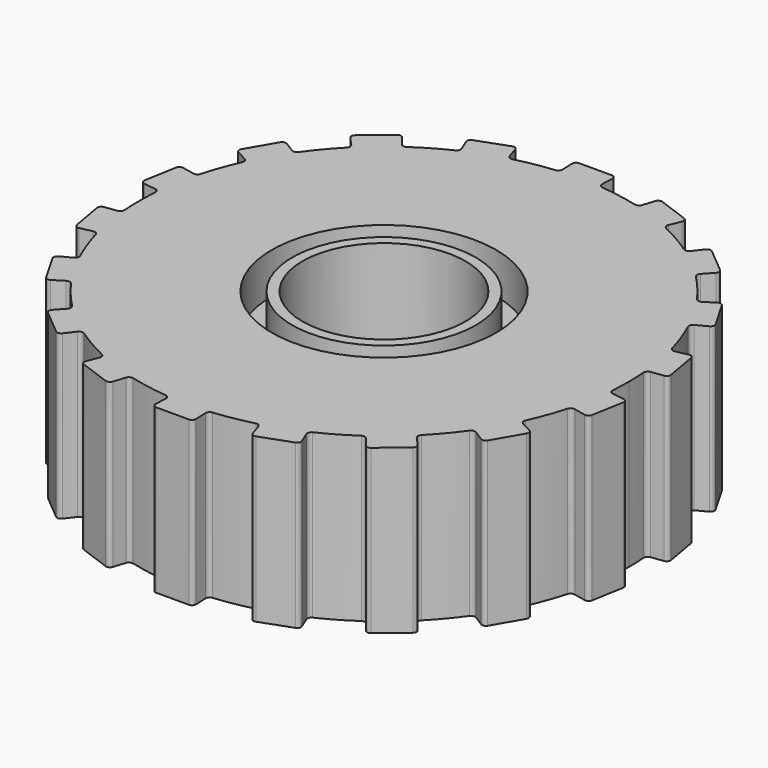
from build123d import *

# Parameters (mm, degrees)
F0_W     = 2.25
F0_H     = 2
F3_DEPTH = 25
F5_R     = 1.375
F5_R_2   = 1.125
F6_DEPTH = 0.5
F4_R     = 1.375
F4_R_2   = 1.125
F7_DEPTH = 0.5


with BuildPart() as f1:
    # F0 (on Front) → F1 (revolve)
    with BuildSketch(Plane.XZ):
        with Locations((-2.125, 1)):
            Rectangle(F0_W, F0_H)
    revolve(axis=Axis((0, 0, 1), (0, 0, 1)))

    # F2 (on face) → F3 (cut)
    with BuildSketch(Plane.XY.offset(2)):
        with BuildLine():
            Line((-0.2480712081, 3.1903703492), (-0.25, 3.2403703492))
            ThreePointArc((-0.25, 3.2403703492), (-0.5643565774, 3.2006251973), (-0.8733487761, 3.1304571416))
            Line((-0.8733487761, 3.1304571416), (-0.8580602404, 3.0828128249))
            Line((-0.8580602404, 3.0828128249), (-0.8121919363, 2.9398714697))
            ThreePointArc((-0.8121919363, 2.9398714697), (-0.7887137207, 2.9105413826), (-0.7516649064, 2.9043071237))
            ThreePointArc((-0.7516649064, 2.9043071237), (-0.520944533, 2.954423259), (-0.2869975729, 2.9862405116))
            Line((-0.2869975729, 2.9862405116), (-0.2980712081, 3.1903703492))
            Line((-0.2980712081, 3.1903703492), (-0.2480712081, 3.1903703492))
        make_face()
        with BuildLine():
            Line((-0.2422844922, 3.0403615286), (-0.2480712081, 3.1903703492))
            Line((-0.2480712081, 3.1903703492), (-0.2980712081, 3.1903703492))
            Line((-0.2980712081, 3.1903703492), (-0.2869975729, 2.9862405116))
            ThreePointArc((-0.2869975729, 2.9862405116), (-0.2543153176, 3.0047702395), (-0.2422844922, 3.0403615286))
        make_face()
        with BuildLine():
            ThreePointArc((-0.2480712081, 3.1903703492), (-0.2346801134, 3.2256042376), (-0.2, 3.2403703492))
            Line((-0.2, 3.2403703492), (-0.25, 3.2403703492))
            Line((-0.25, 3.2403703492), (-0.2480712081, 3.1903703492))
        make_face()
        with BuildLine():
            Line((-0.2, 3.2403703492), (0, 3.2403703492))
            Line((0, 3.2403703492), (0, 3.25))
            ThreePointArc((0, 3.25), (-0.1250926958, 3.247591695), (-0.25, 3.2403703492))
            Line((-0.25, 3.2403703492), (-0.2, 3.2403703492))
        make_face()
        with BuildLine():
            Line((0, 3.25), (0, 3.2403703492))
            Line((0, 3.2403703492), (0.2, 3.2403703492))
            Line((0.2, 3.2403703492), (0.25, 3.2403703492))
            ThreePointArc((0.25, 3.2403703492), (0.1250926958, 3.247591695), (0, 3.25))
        make_face()
        with BuildLine():
            Line((0.25, 3.2403703492), (0.2, 3.2403703492))
            ThreePointArc((0.2, 3.2403703492), (0.2346801134, 3.2256042376), (0.2480712081, 3.1903703492))
            Line((0.2480712081, 3.1903703492), (0.25, 3.2403703492))
        make_face()
        with BuildLine():
            ThreePointArc((0.8733487761, 3.1304571416), (0.5643565774, 3.2006251973), (0.25, 3.2403703492))
            Line((0.25, 3.2403703492), (0.2480712081, 3.1903703492))
            Line((0.2480712081, 3.1903703492), (0.2980712081, 3.1903703492))
            Line((0.2980712081, 3.1903703492), (0.2869975729, 2.9862405116))
            ThreePointArc((0.2869975729, 2.9862405116), (0.520944533, 2.954423259), (0.7516649064, 2.9043071237))
            ThreePointArc((0.7516649064, 2.9043071237), (0.7887137207, 2.9105413826), (0.8121919363, 2.9398714697))
            Line((0.8121919363, 2.9398714697), (0.8580602404, 3.0828128249))
            Line((0.8580602404, 3.0828128249), (0.8733487761, 3.1304571416))
        make_face()
        with BuildLine():
            Line((0.2980712081, 3.1903703492), (0.2480712081, 3.1903703492))
            Line((0.2480712081, 3.1903703492), (0.2422844922, 3.0403615286))
            ThreePointArc((0.2422844922, 3.0403615286), (0.2543153176, 3.0047702395), (0.2869975729, 2.9862405116))
            Line((0.2869975729, 2.9862405116), (0.2980712081, 3.1903703492))
        make_face()
        with BuildLine():
            Line((-1.9296610226, -2.6108252216), (-1.8913588005, -2.6429646021))
            Line((-1.8913588005, -2.6429646021), (-1.8606969603, -2.6034225764))
            ThreePointArc((-1.8606969603, -2.6034225764), (-1.893603041, -2.6218056711), (-1.9296610226, -2.6108252216))
        make_face()
        with BuildLine():
            Line((-2.2360787999, -2.3537101777), (-2.274381022, -2.3215707972))
            ThreePointArc((-2.274381022, -2.3215707972), (-2.0890597315, -2.4896444401), (-1.8913588005, -2.6429646021))
            Line((-1.8913588005, -2.6429646021), (-1.9296610226, -2.6108252216))
            Line((-1.9296610226, -2.6108252216), (-2.2360787999, -2.3537101777))
        make_face()
        with BuildLine():
            Line((-2.2407641013, -2.2845083786), (-2.274381022, -2.3215707972))
            Line((-2.274381022, -2.3215707972), (-2.2360787999, -2.3537101777))
            ThreePointArc((-2.2360787999, -2.3537101777), (-2.2531538345, -2.3201067328), (-2.2407641013, -2.2845083786))
        make_face()
        with BuildLine():
            Line((-2.6389061658, -1.8100211428), (-2.6812430401, -1.8366915255))
            ThreePointArc((-2.6812430401, -1.8366915255), (-2.4896444401, -2.0890597315), (-2.274381022, -2.3215707972))
            Line((-2.274381022, -2.3215707972), (-2.2407641013, -2.2845083786))
            Line((-2.2407641013, -2.2845083786), (-2.1399074085, -2.1733145845))
            ThreePointArc((-2.1399074085, -2.1733145845), (-2.1262459157, -2.1383168097), (-2.1393712963, -2.1031144659))
            ThreePointArc((-2.1393712963, -2.1031144659), (-2.2981333294, -1.9283628291), (-2.4426613584, -1.7416674447))
            ThreePointArc((-2.4426613584, -1.7416674447), (-2.4750497011, -1.7226286454), (-2.5118880744, -1.7300052895))
            Line((-2.5118880744, -1.7300052895), (-2.6389061658, -1.8100211428))
        make_face()
        with BuildLine():
            Line((-2.7062430401, -1.7933902554), (-2.6812430401, -1.8366915255))
            Line((-2.6812430401, -1.8366915255), (-2.6389061658, -1.8100211428))
            ThreePointArc((-2.6389061658, -1.8100211428), (-2.6761151557, -1.8160410588), (-2.7062430401, -1.7933902554))
        make_face()
        with BuildLine():
            Line((-2.9062430401, -1.4469800938), (-2.9312430401, -1.4036788237))
            ThreePointArc((-2.9312430401, -1.4036788237), (-2.8145825623, -1.625), (-2.6812430401, -1.8366915255))
            Line((-2.6812430401, -1.8366915255), (-2.7062430401, -1.7933902554))
            Line((-2.7062430401, -1.7933902554), (-2.9062430401, -1.4469800938))
        make_face()
        with BuildLine():
            Line((-3.0988243417, -0.7983044463), (-3.1477297981, -0.8088863444))
            ThreePointArc((-3.1477297981, -0.8088863444), (-3.0540010176, -1.1115654658), (-2.9312430401, -1.4036788237))
            Line((-2.9312430401, -1.4036788237), (-2.886977374, -1.3803492064))
            Line((-2.886977374, -1.3803492064), (-2.7541725666, -1.3103562391))
            ThreePointArc((-2.7541725666, -1.3103562391), (-2.7293650187, -1.2821415941), (-2.7296589313, -1.2445730669))
            ThreePointArc((-2.7296589313, -1.2445730669), (-2.8190778624, -1.02606043), (-2.8910362027, -0.8011926578))
            ThreePointArc((-2.8910362027, -0.8011926578), (-2.9149596364, -0.7722245729), (-2.9520993448, -0.7665568853))
            Line((-2.9520993448, -0.7665568853), (-3.0988243417, -0.7983044463))
        make_face()
        with BuildLine():
            Line((-2.886977374, -1.3803492064), (-2.9312430401, -1.4036788237))
            Line((-2.9312430401, -1.4036788237), (-2.9062430401, -1.4469800938))
            ThreePointArc((-2.9062430401, -1.4469800938), (-2.910795269, -1.4095631789), (-2.886977374, -1.3803492064))
        make_face()
        with BuildLine():
            Line((-3.2258714781, -0.3657228555), (-3.2345538869, -0.3164824679))
            ThreePointArc((-3.2345538869, -0.3164824679), (-3.2006251973, -0.5643565774), (-3.1477297981, -0.8088863444))
            Line((-3.1477297981, -0.8088863444), (-3.156412207, -0.7596459567))
            Line((-3.156412207, -0.7596459567), (-3.2258714781, -0.3657228555))
        make_face()
        with BuildLine():
            Line((-3.156412207, -0.7596459567), (-3.1477297981, -0.8088863444))
            Line((-3.1477297981, -0.8088863444), (-3.0988243417, -0.7983044463))
            ThreePointArc((-3.0988243417, -0.7983044463), (-3.1358482874, -0.7912350929), (-3.156412207, -0.7596459567))
        make_face()
        with BuildLine():
            Line((-3.1849785681, -0.3096995482), (-3.2345538869, -0.3164824679))
            Line((-3.2345538869, -0.3164824679), (-3.2258714781, -0.3657228555))
            ThreePointArc((-3.2258714781, -0.3657228555), (-3.2173518354, -0.3290055026), (-3.1849785681, -0.3096995482))
        make_face()
        with BuildLine():
            Line((-3.1849785681, 0.3096995482), (-3.2345538869, 0.3164824679))
            ThreePointArc((-3.2345538869, 0.3164824679), (-3.25, 0), (-3.2345538869, -0.3164824679))
            Line((-3.2345538869, -0.3164824679), (-3.1849785681, -0.3096995482))
            Line((-3.1849785681, -0.3096995482), (-3.0362438659, -0.2893495925))
            ThreePointArc((-3.0362438659, -0.2893495925), (-3.0032824193, -0.2713211799), (-2.9907094137, -0.2359177881))
            ThreePointArc((-2.9907094137, -0.2359177881), (-3, 0), (-2.9907094137, 0.2359177881))
            ThreePointArc((-2.9907094137, 0.2359177881), (-3.0032824193, 0.2713211799), (-3.0362438659, 0.2893495925))
            Line((-3.0362438659, 0.2893495925), (-3.1849785681, 0.3096995482))
        make_face()
        with BuildLine():
            Line((-3.2258714781, 0.3657228555), (-3.2345538869, 0.3164824679))
            Line((-3.2345538869, 0.3164824679), (-3.1849785681, 0.3096995482))
            ThreePointArc((-3.1849785681, 0.3096995482), (-3.2173518354, 0.3290055026), (-3.2258714781, 0.3657228555))
        make_face()
        with BuildLine():
            Line((-3.156412207, 0.7596459567), (-3.1477297981, 0.8088863444))
            ThreePointArc((-3.1477297981, 0.8088863444), (-3.2006251973, 0.5643565774), (-3.2345538869, 0.3164824679))
            Line((-3.2345538869, 0.3164824679), (-3.2258714781, 0.3657228555))
            Line((-3.2258714781, 0.3657228555), (-3.156412207, 0.7596459567))
        make_face()
        with BuildLine():
            Line((-3.0988243417, 0.7983044463), (-3.1477297981, 0.8088863444))
            Line((-3.1477297981, 0.8088863444), (-3.156412207, 0.7596459567))
            ThreePointArc((-3.156412207, 0.7596459567), (-3.1358482874, 0.7912350929), (-3.0988243417, 0.7983044463))
        make_face()
        with BuildLine():
            Line((-2.886977374, 1.3803492064), (-2.9312430401, 1.4036788237))
            ThreePointArc((-2.9312430401, 1.4036788237), (-3.0540010176, 1.1115654658), (-3.1477297981, 0.8088863444))
            Line((-3.1477297981, 0.8088863444), (-3.0988243417, 0.7983044463))
            Line((-3.0988243417, 0.7983044463), (-2.9520993448, 0.7665568853))
            ThreePointArc((-2.9520993448, 0.7665568853), (-2.9149596364, 0.7722245729), (-2.8910362027, 0.8011926578))
            ThreePointArc((-2.8910362027, 0.8011926578), (-2.8190778624, 1.02606043), (-2.7296589313, 1.2445730669))
            ThreePointArc((-2.7296589313, 1.2445730669), (-2.7293650187, 1.2821415941), (-2.7541725666, 1.3103562391))
            Line((-2.7541725666, 1.3103562391), (-2.886977374, 1.3803492064))
        make_face()
        with BuildLine():
            Line((-2.9062430401, 1.4469800938), (-2.9312430401, 1.4036788237))
            Line((-2.9312430401, 1.4036788237), (-2.886977374, 1.3803492064))
            ThreePointArc((-2.886977374, 1.3803492064), (-2.910795269, 1.4095631789), (-2.9062430401, 1.4469800938))
        make_face()
        with BuildLine():
            Line((-2.7062430401, 1.7933902554), (-2.6812430401, 1.8366915255))
            ThreePointArc((-2.6812430401, 1.8366915255), (-2.8145825623, 1.625), (-2.9312430401, 1.4036788237))
            Line((-2.9312430401, 1.4036788237), (-2.9062430401, 1.4469800938))
            Line((-2.9062430401, 1.4469800938), (-2.7062430401, 1.7933902554))
        make_face()
        with BuildLine():
            Line((-2.6389061658, 1.8100211428), (-2.6812430401, 1.8366915255))
            Line((-2.6812430401, 1.8366915255), (-2.7062430401, 1.7933902554))
            ThreePointArc((-2.7062430401, 1.7933902554), (-2.6761151557, 1.8160410588), (-2.6389061658, 1.8100211428))
        make_face()
        with BuildLine():
            Line((-1.9296610226, 2.6108252216), (-1.8913588005, 2.6429646021))
            ThreePointArc((-1.8913588005, 2.6429646021), (-2.0890597315, 2.4896444401), (-2.274381022, 2.3215707972))
            Line((-2.274381022, 2.3215707972), (-2.2360787999, 2.3537101777))
            Line((-2.2360787999, 2.3537101777), (-1.9296610226, 2.6108252216))
        make_face()
        with BuildLine():
            Line((-2.2360787999, 2.3537101777), (-2.274381022, 2.3215707972))
            Line((-2.274381022, 2.3215707972), (-2.2407641013, 2.2845083786))
            ThreePointArc((-2.2407641013, 2.2845083786), (-2.2531538345, 2.3201067328), (-2.2360787999, 2.3537101777))
        make_face()
        with BuildLine():
            Line((-2.2407641013, 2.2845083786), (-2.274381022, 2.3215707972))
            ThreePointArc((-2.274381022, 2.3215707972), (-2.4896444401, 2.0890597315), (-2.6812430401, 1.8366915255))
            Line((-2.6812430401, 1.8366915255), (-2.6389061658, 1.8100211428))
            Line((-2.6389061658, 1.8100211428), (-2.5118880744, 1.7300052895))
            ThreePointArc((-2.5118880744, 1.7300052895), (-2.4750497011, 1.7226286454), (-2.4426613584, 1.7416674447))
            ThreePointArc((-2.4426613584, 1.7416674447), (-2.2981333294, 1.9283628291), (-2.1393712963, 2.1031144659))
            ThreePointArc((-2.1393712963, 2.1031144659), (-2.1262459157, 2.1383168097), (-2.1399074085, 2.1733145845))
            Line((-2.1399074085, 2.1733145845), (-2.2407641013, 2.2845083786))
        make_face()
        with BuildLine():
            Line((-1.8606969603, 2.6034225764), (-1.8913588005, 2.6429646021))
            Line((-1.8913588005, 2.6429646021), (-1.9296610226, 2.6108252216))
            ThreePointArc((-1.9296610226, 2.6108252216), (-1.893603041, 2.6218056711), (-1.8606969603, 2.6034225764))
        make_face()
        with BuildLine():
            Line((-1.3242816078, 2.9131221246), (-1.3431950865, 2.9594470699))
            ThreePointArc((-1.3431950865, 2.9594470699), (-1.625, 2.8145825623), (-1.8913588005, 2.6429646021))
            Line((-1.8913588005, 2.6429646021), (-1.8606969603, 2.6034225764))
            Line((-1.8606969603, 2.6034225764), (-1.7687060306, 2.4847895237))
            ThreePointArc((-1.7687060306, 2.4847895237), (-1.736612244, 2.4652582799), (-1.6996655045, 2.4720714336))
            ThreePointArc((-1.6996655045, 2.4720714336), (-1.5, 2.5980762114), (-1.2910439092, 2.7079892216))
            ThreePointArc((-1.2910439092, 2.7079892216), (-1.2666701753, 2.7365794598), (-1.2675378353, 2.7741391162))
            Line((-1.2675378353, 2.7741391162), (-1.3242816078, 2.9131221246))
        make_face()
        with BuildLine():
            Line((-1.2962104554, 2.9765480771), (-1.3431950865, 2.9594470699))
            Line((-1.3431950865, 2.9594470699), (-1.3242816078, 2.9131221246))
            ThreePointArc((-1.3242816078, 2.9131221246), (-1.3237487944, 2.9508111737), (-1.2962104554, 2.9765480771))
        make_face()
        with BuildLine():
            Line((-0.8580602404, 3.0828128249), (-0.8733487761, 3.1304571416))
            Line((-0.8733487761, 3.1304571416), (-0.9203334071, 3.1133561344))
            ThreePointArc((-0.9203334071, 3.1133561344), (-0.8826944529, 3.1113418257), (-0.8580602404, 3.0828128249))
        make_face()
        with BuildLine():
            Line((-0.9203334071, 3.1133561344), (-0.8733487761, 3.1304571416))
            ThreePointArc((-0.8733487761, 3.1304571416), (-1.1115654658, 3.0540010176), (-1.3431950865, 2.9594470699))
            Line((-1.3431950865, 2.9594470699), (-1.2962104554, 2.9765480771))
            Line((-1.2962104554, 2.9765480771), (-0.9203334071, 3.1133561344))
        make_face()
        with BuildLine():
            Line((3.2258714781, -0.3657228555), (3.2345538869, -0.3164824679))
            Line((3.2345538869, -0.3164824679), (3.1849785681, -0.3096995482))
            ThreePointArc((3.1849785681, -0.3096995482), (3.2173518354, -0.3290055026), (3.2258714781, -0.3657228555))
        make_face()
        with BuildLine():
            ThreePointArc((3.1477297981, -0.8088863444), (3.2006251973, -0.5643565774), (3.2345538869, -0.3164824679))
            Line((3.2345538869, -0.3164824679), (3.2258714781, -0.3657228555))
            Line((3.2258714781, -0.3657228555), (3.156412207, -0.7596459567))
            Line((3.156412207, -0.7596459567), (3.1477297981, -0.8088863444))
        make_face()
        with BuildLine():
            Line((3.0988243417, -0.7983044463), (3.1477297981, -0.8088863444))
            Line((3.1477297981, -0.8088863444), (3.156412207, -0.7596459567))
            ThreePointArc((3.156412207, -0.7596459567), (3.1358482874, -0.7912350929), (3.0988243417, -0.7983044463))
        make_face()
        with BuildLine():
            ThreePointArc((2.9312430401, -1.4036788237), (3.0540010176, -1.1115654658), (3.1477297981, -0.8088863444))
            Line((3.1477297981, -0.8088863444), (3.0988243417, -0.7983044463))
            Line((3.0988243417, -0.7983044463), (2.9520993448, -0.7665568853))
            ThreePointArc((2.9520993448, -0.7665568853), (2.9149596364, -0.7722245729), (2.8910362027, -0.8011926578))
            ThreePointArc((2.8910362027, -0.8011926578), (2.8190778624, -1.02606043), (2.7296589313, -1.2445730669))
            ThreePointArc((2.7296589313, -1.2445730669), (2.7293650187, -1.2821415941), (2.7541725666, -1.3103562391))
            Line((2.7541725666, -1.3103562391), (2.886977374, -1.3803492064))
            Line((2.886977374, -1.3803492064), (2.9312430401, -1.4036788237))
        make_face()
        with BuildLine():
            Line((2.9062430401, -1.4469800938), (2.9312430401, -1.4036788237))
            Line((2.9312430401, -1.4036788237), (2.886977374, -1.3803492064))
            ThreePointArc((2.886977374, -1.3803492064), (2.910795269, -1.4095631789), (2.9062430401, -1.4469800938))
        make_face()
        with BuildLine():
            ThreePointArc((2.6812430401, -1.8366915255), (2.8145825623, -1.625), (2.9312430401, -1.4036788237))
            Line((2.9312430401, -1.4036788237), (2.9062430401, -1.4469800938))
            Line((2.9062430401, -1.4469800938), (2.7062430401, -1.7933902554))
            Line((2.7062430401, -1.7933902554), (2.6812430401, -1.8366915255))
        make_face()
        with BuildLine():
            Line((2.6389061658, -1.8100211428), (2.6812430401, -1.8366915255))
            Line((2.6812430401, -1.8366915255), (2.7062430401, -1.7933902554))
            ThreePointArc((2.7062430401, -1.7933902554), (2.6761151557, -1.8160410588), (2.6389061658, -1.8100211428))
        make_face()
        with BuildLine():
            ThreePointArc((2.274381022, -2.3215707972), (2.4896444401, -2.0890597315), (2.6812430401, -1.8366915255))
            Line((2.6812430401, -1.8366915255), (2.6389061658, -1.8100211428))
            Line((2.6389061658, -1.8100211428), (2.5118880744, -1.7300052895))
            ThreePointArc((2.5118880744, -1.7300052895), (2.4750497011, -1.7226286454), (2.4426613584, -1.7416674447))
            ThreePointArc((2.4426613584, -1.7416674447), (2.2981333294, -1.9283628291), (2.1393712963, -2.1031144659))
            ThreePointArc((2.1393712963, -2.1031144659), (2.1262459157, -2.1383168097), (2.1399074085, -2.1733145845))
            Line((2.1399074085, -2.1733145845), (2.2407641013, -2.2845083786))
            Line((2.2407641013, -2.2845083786), (2.274381022, -2.3215707972))
        make_face()
        with BuildLine():
            Line((2.2360787999, -2.3537101777), (2.274381022, -2.3215707972))
            Line((2.274381022, -2.3215707972), (2.2407641013, -2.2845083786))
            ThreePointArc((2.2407641013, -2.2845083786), (2.2531538345, -2.3201067328), (2.2360787999, -2.3537101777))
        make_face()
        with BuildLine():
            ThreePointArc((1.8913588005, -2.6429646021), (2.0890597315, -2.4896444401), (2.274381022, -2.3215707972))
            Line((2.274381022, -2.3215707972), (2.2360787999, -2.3537101777))
            Line((2.2360787999, -2.3537101777), (1.9296610226, -2.6108252216))
            Line((1.9296610226, -2.6108252216), (1.8913588005, -2.6429646021))
        make_face()
        with BuildLine():
            Line((1.2962104554, -2.9765480771), (1.3431950865, -2.9594470699))
            Line((1.3431950865, -2.9594470699), (1.3242816078, -2.9131221246))
            ThreePointArc((1.3242816078, -2.9131221246), (1.3237487944, -2.9508111737), (1.2962104554, -2.9765480771))
        make_face()
        with BuildLine():
            ThreePointArc((0.8733487761, -3.1304571416), (1.1115654658, -3.0540010176), (1.3431950865, -2.9594470699))
            Line((1.3431950865, -2.9594470699), (1.2962104554, -2.9765480771))
            Line((1.2962104554, -2.9765480771), (0.9203334071, -3.1133561344))
            Line((0.9203334071, -3.1133561344), (0.8733487761, -3.1304571416))
        make_face()
        with BuildLine():
            Line((0.2, -3.2403703492), (0.25, -3.2403703492))
            Line((0.25, -3.2403703492), (0.2480712081, -3.1903703492))
            ThreePointArc((0.2480712081, -3.1903703492), (0.2346801134, -3.2256042376), (0.2, -3.2403703492))
        make_face()
        with BuildLine():
            Line((-0.2, -3.2403703492), (-0.25, -3.2403703492))
            ThreePointArc((-0.25, -3.2403703492), (0, -3.25), (0.25, -3.2403703492))
            Line((0.25, -3.2403703492), (0.2, -3.2403703492))
            Line((0.2, -3.2403703492), (-0.2, -3.2403703492))
        make_face()
        with BuildLine():
            Line((-0.2480712081, -3.1903703492), (-0.25, -3.2403703492))
            Line((-0.25, -3.2403703492), (-0.2, -3.2403703492))
            ThreePointArc((-0.2, -3.2403703492), (-0.2346801134, -3.2256042376), (-0.2480712081, -3.1903703492))
        make_face()
        with BuildLine():
            Line((-0.8580602404, -3.0828128249), (-0.8733487761, -3.1304571416))
            ThreePointArc((-0.8733487761, -3.1304571416), (-0.5643565774, -3.2006251973), (-0.25, -3.2403703492))
            Line((-0.25, -3.2403703492), (-0.2480712081, -3.1903703492))
            Line((-0.2480712081, -3.1903703492), (-0.2422844922, -3.0403615286))
            ThreePointArc((-0.2422844922, -3.0403615286), (-0.2543153176, -3.0047702395), (-0.2869975729, -2.9862405116))
            ThreePointArc((-0.2869975729, -2.9862405116), (-0.520944533, -2.954423259), (-0.7516649064, -2.9043071237))
            ThreePointArc((-0.7516649064, -2.9043071237), (-0.7887137207, -2.9105413826), (-0.8121919363, -2.9398714697))
            Line((-0.8121919363, -2.9398714697), (-0.8580602404, -3.0828128249))
        make_face()
        with BuildLine():
            ThreePointArc((0.25, -3.2403703492), (0.5643565774, -3.2006251973), (0.8733487761, -3.1304571416))
            Line((0.8733487761, -3.1304571416), (0.8580602404, -3.0828128249))
            Line((0.8580602404, -3.0828128249), (0.8121919363, -2.9398714697))
            ThreePointArc((0.8121919363, -2.9398714697), (0.7887137207, -2.9105413826), (0.7516649064, -2.9043071237))
            ThreePointArc((0.7516649064, -2.9043071237), (0.520944533, -2.954423259), (0.2869975729, -2.9862405116))
            ThreePointArc((0.2869975729, -2.9862405116), (0.2543153176, -3.0047702395), (0.2422844922, -3.0403615286))
            Line((0.2422844922, -3.0403615286), (0.2480712081, -3.1903703492))
            Line((0.2480712081, -3.1903703492), (0.25, -3.2403703492))
        make_face()
        with BuildLine():
            ThreePointArc((1.3431950865, -2.9594470699), (1.625, -2.8145825623), (1.8913588005, -2.6429646021))
            Line((1.8913588005, -2.6429646021), (1.8606969603, -2.6034225764))
            Line((1.8606969603, -2.6034225764), (1.7687060306, -2.4847895237))
            ThreePointArc((1.7687060306, -2.4847895237), (1.736612244, -2.4652582799), (1.6996655045, -2.4720714336))
            ThreePointArc((1.6996655045, -2.4720714336), (1.5, -2.5980762114), (1.2910439092, -2.7079892216))
            ThreePointArc((1.2910439092, -2.7079892216), (1.2666701753, -2.7365794598), (1.2675378353, -2.7741391162))
            Line((1.2675378353, -2.7741391162), (1.3242816078, -2.9131221246))
            Line((1.3242816078, -2.9131221246), (1.3431950865, -2.9594470699))
        make_face()
        with BuildLine():
            Line((0.8580602404, -3.0828128249), (0.8733487761, -3.1304571416))
            Line((0.8733487761, -3.1304571416), (0.9203334071, -3.1133561344))
            ThreePointArc((0.9203334071, -3.1133561344), (0.8826944529, -3.1113418257), (0.8580602404, -3.0828128249))
        make_face()
        with BuildLine():
            Line((1.8606969603, -2.6034225764), (1.8913588005, -2.6429646021))
            Line((1.8913588005, -2.6429646021), (1.9296610226, -2.6108252216))
            ThreePointArc((1.9296610226, -2.6108252216), (1.893603041, -2.6218056711), (1.8606969603, -2.6034225764))
        make_face()
        with BuildLine():
            Line((-0.9203334071, -3.1133561344), (-0.8733487761, -3.1304571416))
            Line((-0.8733487761, -3.1304571416), (-0.8580602404, -3.0828128249))
            ThreePointArc((-0.8580602404, -3.0828128249), (-0.8826944529, -3.1113418257), (-0.9203334071, -3.1133561344))
        make_face()
        with BuildLine():
            Line((-1.2962104554, -2.9765480771), (-1.3431950865, -2.9594470699))
            ThreePointArc((-1.3431950865, -2.9594470699), (-1.1115654658, -3.0540010176), (-0.8733487761, -3.1304571416))
            Line((-0.8733487761, -3.1304571416), (-0.9203334071, -3.1133561344))
            Line((-0.9203334071, -3.1133561344), (-1.2962104554, -2.9765480771))
        make_face()
        with BuildLine():
            Line((-1.3242816078, -2.9131221246), (-1.3431950865, -2.9594470699))
            Line((-1.3431950865, -2.9594470699), (-1.2962104554, -2.9765480771))
            ThreePointArc((-1.2962104554, -2.9765480771), (-1.3237487944, -2.9508111737), (-1.3242816078, -2.9131221246))
        make_face()
        with BuildLine():
            Line((-1.8606969603, -2.6034225764), (-1.8913588005, -2.6429646021))
            ThreePointArc((-1.8913588005, -2.6429646021), (-1.625, -2.8145825623), (-1.3431950865, -2.9594470699))
            Line((-1.3431950865, -2.9594470699), (-1.3242816078, -2.9131221246))
            Line((-1.3242816078, -2.9131221246), (-1.2675378353, -2.7741391162))
            ThreePointArc((-1.2675378353, -2.7741391162), (-1.2666701753, -2.7365794598), (-1.2910439092, -2.7079892216))
            ThreePointArc((-1.2910439092, -2.7079892216), (-1.5, -2.5980762114), (-1.6996655045, -2.4720714336))
            ThreePointArc((-1.6996655045, -2.4720714336), (-1.736612244, -2.4652582799), (-1.7687060306, -2.4847895237))
            Line((-1.7687060306, -2.4847895237), (-1.8606969603, -2.6034225764))
        make_face()
        with BuildLine():
            ThreePointArc((3.25, 0), (3.2461361749, 0.158429586), (3.2345538869, 0.3164824679))
            Line((3.2345538869, 0.3164824679), (3.1849785681, 0.3096995482))
            Line((3.1849785681, 0.3096995482), (3.0362438659, 0.2893495925))
            ThreePointArc((3.0362438659, 0.2893495925), (3.0032824193, 0.2713211799), (2.9907094137, 0.2359177881))
            ThreePointArc((2.9907094137, 0.2359177881), (2.9976764536, 0.1180503258), (3, 0))
            ThreePointArc((3, 0), (2.9976764536, -0.1180503258), (2.9907094137, -0.2359177881))
            ThreePointArc((2.9907094137, -0.2359177881), (3.0032824193, -0.2713211799), (3.0362438659, -0.2893495925))
            Line((3.0362438659, -0.2893495925), (3.1849785681, -0.3096995482))
            Line((3.1849785681, -0.3096995482), (3.2345538869, -0.3164824679))
            ThreePointArc((3.2345538869, -0.3164824679), (3.2461361749, -0.158429586), (3.25, 0))
        make_face()
        with BuildLine():
            Line((3.1849785681, 0.3096995482), (3.2345538869, 0.3164824679))
            Line((3.2345538869, 0.3164824679), (3.2258714781, 0.3657228555))
            ThreePointArc((3.2258714781, 0.3657228555), (3.2173518354, 0.3290055026), (3.1849785681, 0.3096995482))
        make_face()
        with BuildLine():
            ThreePointArc((3.2345538869, 0.3164824679), (3.2006251973, 0.5643565774), (3.1477297981, 0.8088863444))
            Line((3.1477297981, 0.8088863444), (3.156412207, 0.7596459567))
            Line((3.156412207, 0.7596459567), (3.2258714781, 0.3657228555))
            Line((3.2258714781, 0.3657228555), (3.2345538869, 0.3164824679))
        make_face()
        with BuildLine():
            Line((3.156412207, 0.7596459567), (3.1477297981, 0.8088863444))
            Line((3.1477297981, 0.8088863444), (3.0988243417, 0.7983044463))
            ThreePointArc((3.0988243417, 0.7983044463), (3.1358482874, 0.7912350929), (3.156412207, 0.7596459567))
        make_face()
        with BuildLine():
            ThreePointArc((3.1477297981, 0.8088863444), (3.0540010176, 1.1115654658), (2.9312430401, 1.4036788237))
            Line((2.9312430401, 1.4036788237), (2.886977374, 1.3803492064))
            Line((2.886977374, 1.3803492064), (2.7541725666, 1.3103562391))
            ThreePointArc((2.7541725666, 1.3103562391), (2.7293650187, 1.2821415941), (2.7296589313, 1.2445730669))
            ThreePointArc((2.7296589313, 1.2445730669), (2.8190778624, 1.02606043), (2.8910362027, 0.8011926578))
            ThreePointArc((2.8910362027, 0.8011926578), (2.9149596364, 0.7722245729), (2.9520993448, 0.7665568853))
            Line((2.9520993448, 0.7665568853), (3.0988243417, 0.7983044463))
            Line((3.0988243417, 0.7983044463), (3.1477297981, 0.8088863444))
        make_face()
        with BuildLine():
            ThreePointArc((2.9312430401, 1.4036788237), (2.8145825623, 1.625), (2.6812430401, 1.8366915255))
            Line((2.6812430401, 1.8366915255), (2.7062430401, 1.7933902554))
            Line((2.7062430401, 1.7933902554), (2.9062430401, 1.4469800938))
            Line((2.9062430401, 1.4469800938), (2.9312430401, 1.4036788237))
        make_face()
        with BuildLine():
            Line((2.7062430401, 1.7933902554), (2.6812430401, 1.8366915255))
            Line((2.6812430401, 1.8366915255), (2.6389061658, 1.8100211428))
            ThreePointArc((2.6389061658, 1.8100211428), (2.6761151557, 1.8160410588), (2.7062430401, 1.7933902554))
        make_face()
        with BuildLine():
            Line((2.886977374, 1.3803492064), (2.9312430401, 1.4036788237))
            Line((2.9312430401, 1.4036788237), (2.9062430401, 1.4469800938))
            ThreePointArc((2.9062430401, 1.4469800938), (2.910795269, 1.4095631789), (2.886977374, 1.3803492064))
        make_face()
        with BuildLine():
            ThreePointArc((1.3431950865, 2.9594470699), (1.1115654658, 3.0540010176), (0.8733487761, 3.1304571416))
            Line((0.8733487761, 3.1304571416), (0.9203334071, 3.1133561344))
            Line((0.9203334071, 3.1133561344), (1.2962104554, 2.9765480771))
            Line((1.2962104554, 2.9765480771), (1.3431950865, 2.9594470699))
        make_face()
        with BuildLine():
            Line((0.9203334071, 3.1133561344), (0.8733487761, 3.1304571416))
            Line((0.8733487761, 3.1304571416), (0.8580602404, 3.0828128249))
            ThreePointArc((0.8580602404, 3.0828128249), (0.8826944529, 3.1113418257), (0.9203334071, 3.1133561344))
        make_face()
        with BuildLine():
            Line((1.3242816078, 2.9131221246), (1.3431950865, 2.9594470699))
            Line((1.3431950865, 2.9594470699), (1.2962104554, 2.9765480771))
            ThreePointArc((1.2962104554, 2.9765480771), (1.3237487944, 2.9508111737), (1.3242816078, 2.9131221246))
        make_face()
        with BuildLine():
            ThreePointArc((1.8913588005, 2.6429646021), (1.625, 2.8145825623), (1.3431950865, 2.9594470699))
            Line((1.3431950865, 2.9594470699), (1.3242816078, 2.9131221246))
            Line((1.3242816078, 2.9131221246), (1.2675378353, 2.7741391162))
            ThreePointArc((1.2675378353, 2.7741391162), (1.2666701753, 2.7365794598), (1.2910439092, 2.7079892216))
            ThreePointArc((1.2910439092, 2.7079892216), (1.5, 2.5980762114), (1.6996655045, 2.4720714336))
            ThreePointArc((1.6996655045, 2.4720714336), (1.736612244, 2.4652582799), (1.7687060306, 2.4847895237))
            Line((1.7687060306, 2.4847895237), (1.8606969603, 2.6034225764))
            Line((1.8606969603, 2.6034225764), (1.8913588005, 2.6429646021))
        make_face()
        with BuildLine():
            ThreePointArc((2.274381022, 2.3215707972), (2.0890597315, 2.4896444401), (1.8913588005, 2.6429646021))
            Line((1.8913588005, 2.6429646021), (1.9296610226, 2.6108252216))
            Line((1.9296610226, 2.6108252216), (2.2360787999, 2.3537101777))
            Line((2.2360787999, 2.3537101777), (2.274381022, 2.3215707972))
        make_face()
        with BuildLine():
            Line((1.9296610226, 2.6108252216), (1.8913588005, 2.6429646021))
            Line((1.8913588005, 2.6429646021), (1.8606969603, 2.6034225764))
            ThreePointArc((1.8606969603, 2.6034225764), (1.893603041, 2.6218056711), (1.9296610226, 2.6108252216))
        make_face()
        with BuildLine():
            Line((2.2407641013, 2.2845083786), (2.274381022, 2.3215707972))
            Line((2.274381022, 2.3215707972), (2.2360787999, 2.3537101777))
            ThreePointArc((2.2360787999, 2.3537101777), (2.2531538345, 2.3201067328), (2.2407641013, 2.2845083786))
        make_face()
        with BuildLine():
            ThreePointArc((2.6812430401, 1.8366915255), (2.4896444401, 2.0890597315), (2.274381022, 2.3215707972))
            Line((2.274381022, 2.3215707972), (2.2407641013, 2.2845083786))
            Line((2.2407641013, 2.2845083786), (2.1399074085, 2.1733145845))
            ThreePointArc((2.1399074085, 2.1733145845), (2.1262459157, 2.1383168097), (2.1393712963, 2.1031144659))
            ThreePointArc((2.1393712963, 2.1031144659), (2.2981333294, 1.9283628291), (2.4426613584, 1.7416674447))
            ThreePointArc((2.4426613584, 1.7416674447), (2.4750497011, 1.7226286454), (2.5118880744, 1.7300052895))
            Line((2.5118880744, 1.7300052895), (2.6389061658, 1.8100211428))
            Line((2.6389061658, 1.8100211428), (2.6812430401, 1.8366915255))
        make_face()
    extrude(amount=-F3_DEPTH, mode=Mode.SUBTRACT)

    # F5 (on face) → F6 (cut)
    with BuildSketch(Plane(origin=(0, 0, 0), x_dir=(1, 0, 0), z_dir=(0, 0, -1))):
        Circle(F5_R)
        Circle(F5_R_2, mode=Mode.SUBTRACT)
    extrude(amount=-F6_DEPTH, mode=Mode.SUBTRACT)

    # F4 (on face) → F7 (cut)
    with BuildSketch(Plane.XY.offset(2)):
        Circle(F4_R)
        Circle(F4_R_2, mode=Mode.SUBTRACT)
    extrude(amount=-F7_DEPTH, mode=Mode.SUBTRACT)


solid = f1.part
